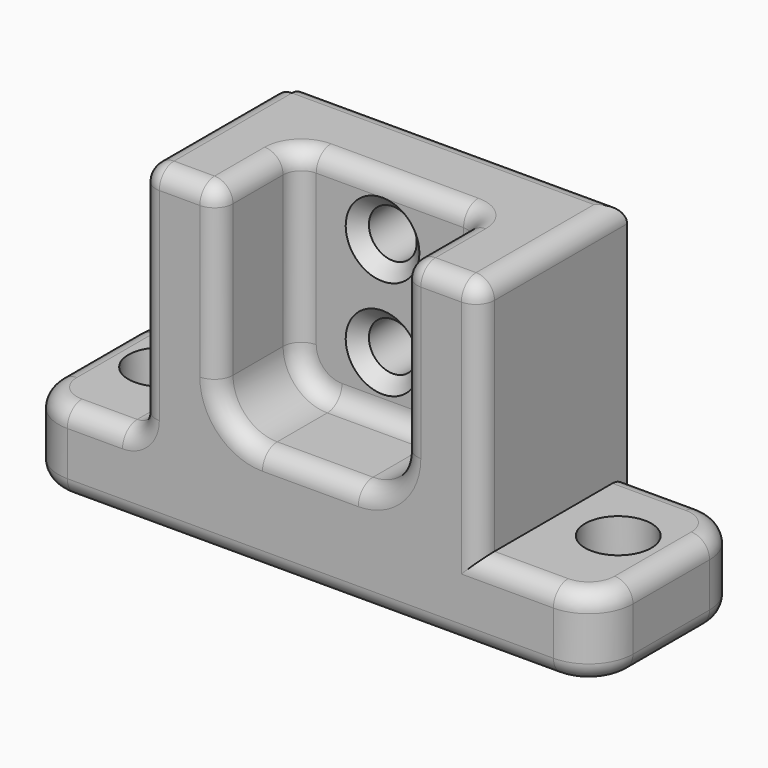
from build123d import *

# Parameters (mm, degrees)
F0_W           = 156
F0_H           = 50
F1_DEPTH       = 87
F2_W           = 32
F2_H           = 65
F3_DEPTH       = 50
F4_W           = 50
F4_H           = 58
F5_DEPTH       = 27
F7_D           = 13
F7_CBORE_D     = 18
F7_CBORE_DEPTH = 10
F9_D           = 13
F9_CSINK_D     = 20
F9_CSINK_ANGLE = 90
F10_R          = 12
F11_T1_DEPTH   = 46
F11_T3_DEPTH   = 26
F11_T5_DEPTH   = 50
F11_T8_ANGLE   = 90
F11_T10_ANGLE  = 90
F11_T11_DEPTH  = 57.5
F11_T13_DEPTH  = 28.5
F11_T15_DEPTH  = 46
F11_T17_DEPTH  = 75
F11_T19_DEPTH  = 117
F11_T21_DEPTH  = 132
F11_T23_DEPTH  = 20
F11_T25_DEPTH  = 60
F11_T27_DEPTH  = 58.5
F11_T29_DEPTH  = 26
F11_T31_DEPTH  = 26
F11_S35_W      = 5
F11_S35_H      = 5
F11_T36_DEPTH  = 5
F11_T40_ANGLE  = 90
F11_T42_ANGLE  = 90
F11_T44_ANGLE  = 90
F11_T46_ANGLE  = 90
F11_T48_ANGLE  = 90
F11_T50_ANGLE  = 90
F11_T52_ANGLE  = 90
F11_T54_ANGLE  = 90
F11_T59_DEPTH  = 72.5
F11_T63_DEPTH  = 32.5
F11_T66_DEPTH  = 17
F11_T68_DEPTH  = 40
F11_T70_DEPTH  = 15
F11_T72_DEPTH  = 55
F11_T74_DEPTH  = 26
F11_S78_W      = 5
F11_S78_H      = 5
F11_T79_DEPTH  = 5
F11_S84_W      = 5
F11_S84_H      = 5
F11_T85_DEPTH  = 5
F11_S90_W      = 5
F11_S90_H      = 5
F11_T91_DEPTH  = 5
F11_S96_W      = 5
F11_S96_H      = 5
F11_T97_DEPTH  = 5
F11_T101_ANGLE = 90
F11_T103_ANGLE = 90
F11_T105_ANGLE = 90
F11_T107_ANGLE = 90
F11_T109_ANGLE = 90
F11_T111_ANGLE = 90


# Not quite as in the source:
# - a fillet or chamfer that OpenCascade refuses, or shapes differently, is made with other operations: its cross-section is extruded or revolved along the edge and cut away or added


with BuildPart() as f1:
    # F0 (on Top) → F1 (new body)
    with BuildSketch(Plane.XY):
        with Locations((78, 25)):
            Rectangle(F0_W, F0_H)
    extrude(amount=F1_DEPTH)

    # F2 (on face) → F3 (cut, through all)
    with BuildSketch(Plane.XZ):
        with Locations((16, 54.5)):
            Rectangle(F2_W, F2_H)
        with Locations((140, 54.5)):
            Rectangle(F2_W, F2_H)
    extrude(amount=-F3_DEPTH, mode=Mode.SUBTRACT)

    # F4 (on face) → F5 (cut)
    with BuildSketch(Plane.XZ):
        with Locations((78, 58)):
            Rectangle(F4_W, F4_H)
    extrude(amount=-F5_DEPTH, mode=Mode.SUBTRACT)

    # F7 (through all)
    with Locations(Plane.XY.offset(22)):
        with Locations((16, 27), (140, 27)):
            CounterBoreHole(F7_D / 2, F7_CBORE_D / 2, F7_CBORE_DEPTH)

    # F9 (through all)
    with Locations(Plane.XZ.offset(-27)):
        with Locations((76, 72), (76, 45)):
            CounterSinkHole(F9_D / 2, F9_CSINK_D / 2, counter_sink_angle=F9_CSINK_ANGLE)

    # F10
    f10_edges = [f1.edges().sort_by_distance(p)[0] for p in [
        (53, 13.5, 29),
        (103, 13.5, 29),
        (0, 0, 11),
        (0, 50, 11),
        (156, 50, 11),
        (156, 0, 11),
    ]]
    fillet(f10_edges, radius=F10_R)

    # F11: fillet of radius 5 on 45 edges, made by hand

    # F11_s2 → F11_t1 (join)
    with BuildSketch(Plane.XY.offset(41)):
        with BuildLine():
            ThreePointArc((53, 22), (54.4644660941, 25.5355339059), (58, 27))
            Line((58, 27), (53, 27))
            Line((53, 27), (53, 22))
        make_face()
        with BuildLine():
            ThreePointArc((103, 22), (101.5355339059, 25.5355339059), (98, 27))
            Line((98, 27), (103, 27))
            Line((103, 27), (103, 22))
        make_face()
    extrude(amount=F11_T1_DEPTH)

    # F11_s4 → F11_t3 (join)
    with BuildSketch(Plane.YZ.offset(65)):
        with BuildLine():
            ThreePointArc((22, 29), (25.5355339059, 30.4644660941), (27, 34))
            Line((27, 34), (27, 29))
            Line((27, 29), (22, 29))
        make_face()
    extrude(amount=F11_T3_DEPTH)

    # F11_s6 → F11_t5 (join)
    with BuildSketch(Plane.XZ.offset(-50)):
        with BuildLine():
            ThreePointArc((27, 22), (30.5355339059, 23.4644660941), (32, 27))
            Line((32, 27), (32, 22))
            Line((32, 22), (27, 22))
        make_face()
    extrude(amount=F11_T5_DEPTH)

    # F11_s7 → F11_t8 (revolve)
    with BuildSketch(Plane.YZ.offset(65)):
        with BuildLine():
            ThreePointArc((22, 29), (25.5355339059, 30.4644660941), (27, 34))
            Line((27, 34), (27, 29))
            Line((27, 29), (22, 29))
        make_face()
    revolve(axis=Axis((65, 27, 41), (0, 1, 0)), revolution_arc=F11_T8_ANGLE)

    # F11_s9 → F11_t10 (revolve)
    with BuildSketch(Plane.XY.offset(41)):
        with BuildLine():
            ThreePointArc((103, 22), (101.5355339059, 25.5355339059), (98, 27))
            Line((98, 27), (103, 27))
            Line((103, 27), (103, 22))
        make_face()
    revolve(axis=Axis((91, 27, 41), (0, 1, 0)), revolution_arc=F11_T10_ANGLE)

    # F11_s12 → F11_t11 (cut)
    with BuildSketch(Plane.XZ.offset(-62.5)):
        with BuildLine():
            ThreePointArc((124, 82), (122.5355339059, 85.5355339059), (119, 87))
            Line((119, 87), (124, 87))
            Line((124, 87), (124, 82))
        make_face()
    extrude(amount=F11_T11_DEPTH, mode=Mode.SUBTRACT)

    # F11_s14 → F11_t13 (cut)
    with BuildSketch(Plane.YZ.offset(90.5)):
        with BuildLine():
            ThreePointArc((0, 82), (1.4644660941, 85.5355339059), (5, 87))
            Line((5, 87), (0, 87))
            Line((0, 87), (0, 82))
        make_face()
    extrude(amount=F11_T13_DEPTH, mode=Mode.SUBTRACT)

    # F11_s16 → F11_t15 (cut)
    with BuildSketch(Plane.YZ.offset(19.5)):
        with BuildLine():
            ThreePointArc((0, 82), (1.4644660941, 85.5355339059), (5, 87))
            Line((5, 87), (0, 87))
            Line((0, 87), (0, 82))
        make_face()
    extrude(amount=F11_T15_DEPTH, mode=Mode.SUBTRACT)

    # F11_s18 → F11_t17 (cut)
    with BuildSketch(Plane.XZ.offset(-62.5)):
        with BuildLine():
            ThreePointArc((32, 82), (33.4644660941, 85.5355339059), (37, 87))
            Line((37, 87), (32, 87))
            Line((32, 87), (32, 82))
        make_face()
    extrude(amount=F11_T17_DEPTH, mode=Mode.SUBTRACT)

    # F11_s20 → F11_t19 (cut)
    with BuildSketch(Plane.YZ.offset(19.5)):
        with BuildLine():
            ThreePointArc((50, 82), (48.5355339059, 85.5355339059), (45, 87))
            Line((45, 87), (50, 87))
            Line((50, 87), (50, 82))
        make_face()
    extrude(amount=F11_T19_DEPTH, mode=Mode.SUBTRACT)

    # F11_s22 → F11_t21 (cut)
    with BuildSketch(Plane.YZ.offset(12)):
        with BuildLine():
            ThreePointArc((5, 0), (1.4644660941, 1.4644660941), (0, 5))
            Line((0, 5), (0, 0))
            Line((0, 0), (5, 0))
        make_face()
        with BuildLine():
            ThreePointArc((45, 0), (48.5355339059, 1.4644660941), (50, 5))
            Line((50, 5), (50, 0))
            Line((50, 0), (45, 0))
        make_face()
    extrude(amount=F11_T21_DEPTH, mode=Mode.SUBTRACT)

    # F11_s24 → F11_t23 (cut)
    with BuildSketch(Plane.YZ.offset(124)):
        with BuildLine():
            ThreePointArc((0, 17), (1.4644660941, 20.5355339059), (5, 22))
            Line((5, 22), (0, 22))
            Line((0, 22), (0, 17))
        make_face()
        with BuildLine():
            ThreePointArc((50, 17), (48.5355339059, 20.5355339059), (45, 22))
            Line((45, 22), (50, 22))
            Line((50, 22), (50, 17))
        make_face()
    extrude(amount=F11_T23_DEPTH, mode=Mode.SUBTRACT)

    # F11_s26 → F11_t25 (cut)
    with BuildSketch(Plane.XY.offset(22)):
        with BuildLine():
            ThreePointArc((119, 0), (122.5355339059, 1.4644660941), (124, 5))
            Line((124, 5), (124, 0))
            Line((124, 0), (119, 0))
        make_face()
    extrude(amount=F11_T25_DEPTH, mode=Mode.SUBTRACT)

    # F11_s28 → F11_t27 (cut)
    with BuildSketch(Plane.XY.offset(41)):
        with BuildLine():
            ThreePointArc((48, 0), (51.5355339059, 1.4644660941), (53, 5))
            Line((53, 5), (53, 0))
            Line((53, 0), (48, 0))
        make_face()
        with BuildLine():
            ThreePointArc((108, 0), (104.4644660941, 1.4644660941), (103, 5))
            Line((103, 5), (103, 0))
            Line((103, 0), (108, 0))
        make_face()
    extrude(amount=F11_T27_DEPTH, mode=Mode.SUBTRACT)

    # F11_s30 → F11_t29 (cut)
    with BuildSketch(Plane.YZ.offset(65)):
        with BuildLine():
            ThreePointArc((0, 24), (1.4644660941, 27.5355339059), (5, 29))
            Line((5, 29), (0, 29))
            Line((0, 29), (0, 24))
        make_face()
    extrude(amount=F11_T29_DEPTH, mode=Mode.SUBTRACT)

    # F11_s32 → F11_t31 (cut)
    with BuildSketch(Plane.XZ.offset(-38)):
        with BuildLine():
            ThreePointArc((0, 5), (1.4644660941, 1.4644660941), (5, 0))
            Line((5, 0), (0, 0))
            Line((0, 0), (0, 5))
        make_face()
        with BuildLine():
            ThreePointArc((151, 0), (154.5355339059, 1.4644660941), (156, 5))
            Line((156, 5), (156, 0))
            Line((156, 0), (151, 0))
        make_face()
        with BuildLine():
            ThreePointArc((156, 17), (154.5355339059, 20.5355339059), (151, 22))
            Line((151, 22), (156, 22))
            Line((156, 22), (156, 17))
        make_face()
    extrude(amount=F11_T31_DEPTH, mode=Mode.SUBTRACT)


with BuildPart() as f11_tool34:
    # F11_s35 → F11_t36 (new body)
    with BuildSketch(Plane.XY.offset(82)):
        with Locations((121.5, 2.5)):
            Rectangle(F11_S35_W, F11_S35_H)
    extrude(amount=F11_T36_DEPTH)

    # F11_s37 → F11_t38 (revolve, cut)
    with BuildSketch(Plane(origin=(119, 5, 82), x_dir=(-0.7071067812, 0.7071067812, 0), z_dir=(0.7071067812, 0.7071067812, 0))):
        with BuildLine():
            ThreePointArc((0, -5), (5, 0), (0, 5))
            Line((0, 5), (0, -5))
        make_face()
    revolve(axis=Axis((119, 5, 82), (0, 0, 1)), mode=Mode.SUBTRACT)


with BuildPart() as f1_1:
    add(f1.part)

    # F11_t33: cut F11_tool34
    add(f11_tool34.part, mode=Mode.SUBTRACT)

    # F11_s39 → F11_t40 (revolve, cut)
    with BuildSketch(Plane.YZ.offset(65)):
        with BuildLine():
            ThreePointArc((0, 24), (1.4644660941, 27.5355339059), (5, 29))
            Line((5, 29), (0, 29))
            Line((0, 29), (0, 24))
        make_face()
    revolve(axis=Axis((65, 0, 41), (0, 1, 0)), revolution_arc=F11_T40_ANGLE, mode=Mode.SUBTRACT)

    # F11_s41 → F11_t42 (revolve, cut)
    with BuildSketch(Plane.XY.offset(41)):
        with BuildLine():
            ThreePointArc((108, 0), (104.4644660941, 1.4644660941), (103, 5))
            Line((103, 5), (103, 0))
            Line((103, 0), (108, 0))
        make_face()
    revolve(axis=Axis((91, 0, 41), (0, 1, 0)), revolution_arc=F11_T42_ANGLE, mode=Mode.SUBTRACT)

    # F11_s43 → F11_t44 (revolve, cut)
    with BuildSketch(Plane.XZ.offset(-38)):
        with BuildLine():
            ThreePointArc((5, 0), (1.4644660941, 1.4644660941), (0, 5))
            Line((0, 5), (0, 0))
            Line((0, 0), (5, 0))
        make_face()
    revolve(axis=Axis((12, 38, 0), (0, 0, -1)), revolution_arc=F11_T44_ANGLE, mode=Mode.SUBTRACT)

    # F11_s45 → F11_t46 (revolve, cut)
    with BuildSketch(Plane.XZ.offset(-12)):
        with BuildLine():
            ThreePointArc((5, 0), (1.4644660941, 1.4644660941), (0, 5))
            Line((0, 5), (0, 0))
            Line((0, 0), (5, 0))
        make_face()
    revolve(axis=Axis((12, 12, 0), (0, 0, 1)), revolution_arc=F11_T46_ANGLE, mode=Mode.SUBTRACT)

    # F11_s47 → F11_t48 (revolve, cut)
    with BuildSketch(Plane.YZ.offset(144)):
        with BuildLine():
            ThreePointArc((45, 0), (48.5355339059, 1.4644660941), (50, 5))
            Line((50, 5), (50, 0))
            Line((50, 0), (45, 0))
        make_face()
    revolve(axis=Axis((144, 38, 0), (0, 0, -1)), revolution_arc=F11_T48_ANGLE, mode=Mode.SUBTRACT)

    # F11_s49 → F11_t50 (revolve, cut)
    with BuildSketch(Plane.YZ.offset(144)):
        with BuildLine():
            ThreePointArc((5, 0), (1.4644660941, 1.4644660941), (0, 5))
            Line((0, 5), (0, 0))
            Line((0, 0), (5, 0))
        make_face()
    revolve(axis=Axis((144, 12, 0), (0, 0, 1)), revolution_arc=F11_T50_ANGLE, mode=Mode.SUBTRACT)

    # F11_s51 → F11_t52 (revolve, cut)
    with BuildSketch(Plane.YZ.offset(144)):
        with BuildLine():
            ThreePointArc((50, 17), (48.5355339059, 20.5355339059), (45, 22))
            Line((45, 22), (50, 22))
            Line((50, 22), (50, 17))
        make_face()
    revolve(axis=Axis((144, 38, 22), (0, 0, -1)), revolution_arc=F11_T52_ANGLE, mode=Mode.SUBTRACT)

    # F11_s53 → F11_t54 (revolve, cut)
    with BuildSketch(Plane.YZ.offset(144)):
        with BuildLine():
            ThreePointArc((0, 17), (1.4644660941, 20.5355339059), (5, 22))
            Line((5, 22), (0, 22))
            Line((0, 22), (0, 17))
        make_face()
    revolve(axis=Axis((144, 12, 22), (0, 0, 1)), revolution_arc=F11_T54_ANGLE, mode=Mode.SUBTRACT)


with BuildPart() as f11_tool57:
    # F11_s58 → F11_t59 (new body)
    with BuildSketch(Plane.XY.offset(82)):
        with BuildLine():
            ThreePointArc((119, 0), (122.5355339059, 1.4644660941), (124, 5))
            Line((124, 5), (124, 0))
            Line((124, 0), (119, 0))
        make_face()
    extrude(amount=-F11_T59_DEPTH)

    split(bisect_by=Plane.XY.offset(22), keep=Keep.BOTTOM)


with BuildPart() as f11_tool61:
    # F11_s62 → F11_t63 (new body)
    with BuildSketch(Plane.YZ.offset(111.5)):
        with BuildLine():
            ThreePointArc((0, 17), (1.4644660941, 20.5355339059), (5, 22))
            Line((5, 22), (0, 22))
            Line((0, 22), (0, 17))
        make_face()
    extrude(amount=F11_T63_DEPTH)

    split(bisect_by=Plane.YZ.offset(124), keep=Keep.BOTTOM)


with BuildPart() as f11_tool57_1:
    add(f11_tool57.part)

    # F11_t65: intersect F11_tool61
    add(f11_tool61.part, mode=Mode.INTERSECT)


with BuildPart() as f1_2:
    add(f1_1.part)

    # F11_t55: cut F11_tool57
    add(f11_tool57_1.part, mode=Mode.SUBTRACT)

    # F11_s67 → F11_t66 (cut)
    with BuildSketch(Plane.XZ.offset(-22)):
        with BuildLine():
            ThreePointArc((108, 87), (104.4644660941, 85.5355339059), (103, 82))
            Line((103, 82), (103, 87))
            Line((103, 87), (108, 87))
        make_face()
        with BuildLine():
            ThreePointArc((48, 87), (51.5355339059, 85.5355339059), (53, 82))
            Line((53, 82), (53, 87))
            Line((53, 87), (48, 87))
        make_face()
    extrude(amount=F11_T66_DEPTH, mode=Mode.SUBTRACT)

    # F11_s69 → F11_t68 (cut)
    with BuildSketch(Plane.YZ.offset(58)):
        with BuildLine():
            ThreePointArc((32, 87), (28.4644660941, 85.5355339059), (27, 82))
            Line((27, 82), (27, 87))
            Line((27, 87), (32, 87))
        make_face()
    extrude(amount=F11_T68_DEPTH, mode=Mode.SUBTRACT)

    # F11_s71 → F11_t70 (cut)
    with BuildSketch(Plane.YZ.offset(12)):
        with BuildLine():
            ThreePointArc((0, 17), (1.4644660941, 20.5355339059), (5, 22))
            Line((5, 22), (0, 22))
            Line((0, 22), (0, 17))
        make_face()
        with BuildLine():
            ThreePointArc((50, 17), (48.5355339059, 20.5355339059), (45, 22))
            Line((45, 22), (50, 22))
            Line((50, 22), (50, 17))
        make_face()
    extrude(amount=F11_T70_DEPTH, mode=Mode.SUBTRACT)

    # F11_s73 → F11_t72 (cut)
    with BuildSketch(Plane.XY.offset(27)):
        with BuildLine():
            ThreePointArc((37, 0), (33.4644660941, 1.4644660941), (32, 5))
            Line((32, 5), (32, 0))
            Line((32, 0), (37, 0))
        make_face()
        with BuildLine():
            ThreePointArc((32, 45), (33.4644660941, 48.5355339059), (37, 50))
            Line((37, 50), (32, 50))
            Line((32, 50), (32, 45))
        make_face()
    extrude(amount=F11_T72_DEPTH, mode=Mode.SUBTRACT)

    # F11_s75 → F11_t74 (cut)
    with BuildSketch(Plane.XZ.offset(-38)):
        with BuildLine():
            ThreePointArc((0, 17), (1.4644660941, 20.5355339059), (5, 22))
            Line((5, 22), (0, 22))
            Line((0, 22), (0, 17))
        make_face()
    extrude(amount=F11_T74_DEPTH, mode=Mode.SUBTRACT)


with BuildPart() as f11_tool77:
    # F11_s78 → F11_t79 (new body)
    with BuildSketch(Plane.YZ.offset(37)):
        with Locations((47.5, 84.5)):
            Rectangle(F11_S78_W, F11_S78_H)
    extrude(amount=-F11_T79_DEPTH)

    # F11_s80 → F11_t81 (revolve, cut)
    with BuildSketch(Plane(origin=(37, 45, 82), x_dir=(0, -0.7071067812, -0.7071067812), z_dir=(0, 0.7071067812, -0.7071067812))):
        with BuildLine():
            ThreePointArc((0, -5), (5, 0), (0, 5))
            Line((0, 5), (0, -5))
        make_face()
    revolve(axis=Axis((37, 45, 82), (-1, 0, 0)), mode=Mode.SUBTRACT)


with BuildPart() as f1_3:
    add(f1_2.part)

    # F11_t76: cut F11_tool77
    add(f11_tool77.part, mode=Mode.SUBTRACT)


with BuildPart() as f11_tool83:
    # F11_s84 → F11_t85 (new body)
    with BuildSketch(Plane.XZ.offset(-5)):
        with Locations((34.5, 84.5)):
            Rectangle(F11_S84_W, F11_S84_H)
    extrude(amount=F11_T85_DEPTH)

    # F11_s86 → F11_t87 (revolve, cut)
    with BuildSketch(Plane(origin=(37, 5, 82), x_dir=(0.7071067812, 0, -0.7071067812), z_dir=(-0.7071067812, 0, -0.7071067812))):
        with BuildLine():
            ThreePointArc((0, -5), (5, 0), (0, 5))
            Line((0, 5), (0, -5))
        make_face()
    revolve(axis=Axis((37, 5, 82), (0, -1, 0)), mode=Mode.SUBTRACT)


with BuildPart() as f1_4:
    add(f1_3.part)

    # F11_t82: cut F11_tool83
    add(f11_tool83.part, mode=Mode.SUBTRACT)


with BuildPart() as f11_tool89:
    # F11_s90 → F11_t91 (new body)
    with BuildSketch(Plane.XY.offset(82)):
        with Locations((50.5, 2.5)):
            Rectangle(F11_S90_W, F11_S90_H)
    extrude(amount=F11_T91_DEPTH)

    # F11_s92 → F11_t93 (revolve, cut)
    with BuildSketch(Plane(origin=(48, 5, 82), x_dir=(-0.7071067812, 0.7071067812, 0), z_dir=(0.7071067812, 0.7071067812, 0))):
        with BuildLine():
            ThreePointArc((0, -5), (5, 0), (0, 5))
            Line((0, 5), (0, -5))
        make_face()
    revolve(axis=Axis((48, 5, 82), (0, 0, 1)), mode=Mode.SUBTRACT)


with BuildPart() as f1_5:
    add(f1_4.part)

    # F11_t88: cut F11_tool89
    add(f11_tool89.part, mode=Mode.SUBTRACT)


with BuildPart() as f11_tool95:
    # F11_s96 → F11_t97 (new body)
    with BuildSketch(Plane.XY.offset(82)):
        with Locations((105.5, 2.5)):
            Rectangle(F11_S96_W, F11_S96_H)
    extrude(amount=F11_T97_DEPTH)

    # F11_s98 → F11_t99 (revolve, cut)
    with BuildSketch(Plane(origin=(108, 5, 82), x_dir=(0.7071067812, 0.7071067812, 0), z_dir=(0.7071067812, -0.7071067812, 0))):
        with BuildLine():
            ThreePointArc((0, -5), (5, 0), (0, 5))
            Line((0, 5), (0, -5))
        make_face()
    revolve(axis=Axis((108, 5, 82), (0, 0, 1)), mode=Mode.SUBTRACT)


with BuildPart() as f1_6:
    add(f1_5.part)

    # F11_t94: cut F11_tool95
    add(f11_tool95.part, mode=Mode.SUBTRACT)

    # F11_s100 → F11_t101 (revolve, cut)
    with BuildSketch(Plane.XZ.offset(-38)):
        with BuildLine():
            ThreePointArc((0, 17), (1.4644660941, 20.5355339059), (5, 22))
            Line((5, 22), (0, 22))
            Line((0, 22), (0, 17))
        make_face()
    revolve(axis=Axis((12, 38, 22), (0, 0, -1)), revolution_arc=F11_T101_ANGLE, mode=Mode.SUBTRACT)

    # F11_s102 → F11_t103 (revolve, cut)
    with BuildSketch(Plane.XZ.offset(-12)):
        with BuildLine():
            ThreePointArc((5, 22), (1.4644660941, 20.5355339059), (0, 17))
            Line((0, 17), (0, 22))
            Line((0, 22), (5, 22))
        make_face()
    revolve(axis=Axis((12, 12, 22), (0, 0, 1)), revolution_arc=F11_T103_ANGLE, mode=Mode.SUBTRACT)

    # F11_s104 → F11_t105 (revolve, cut)
    with BuildSketch(Plane.YZ.offset(27)):
        with BuildLine():
            ThreePointArc((45, 22), (48.5355339059, 20.5355339059), (50, 17))
            Line((50, 17), (50, 22))
            Line((50, 22), (45, 22))
        make_face()
    revolve(axis=Axis((27, 50, 27), (0, -1, 0)), revolution_arc=F11_T105_ANGLE, mode=Mode.SUBTRACT)

    # F11_s106 → F11_t107 (revolve, cut)
    with BuildSketch(Plane.YZ.offset(27)):
        with BuildLine():
            ThreePointArc((0, 17), (1.4644660941, 20.5355339059), (5, 22))
            Line((5, 22), (0, 22))
            Line((0, 22), (0, 17))
        make_face()
    revolve(axis=Axis((27, 0, 27), (0, -1, 0)), revolution_arc=F11_T107_ANGLE, mode=Mode.SUBTRACT)

    # F11_s108 → F11_t109 (revolve, cut)
    with BuildSketch(Plane.XZ.offset(-22)):
        with BuildLine():
            ThreePointArc((48, 87), (51.5355339059, 85.5355339059), (53, 82))
            Line((53, 82), (53, 87))
            Line((53, 87), (48, 87))
        make_face()
    revolve(axis=Axis((58, 22, 87), (0, 0, -1)), revolution_arc=F11_T109_ANGLE, mode=Mode.SUBTRACT)

    # F11_s110 → F11_t111 (revolve, cut)
    with BuildSketch(Plane.XZ.offset(-22)):
        with BuildLine():
            ThreePointArc((108, 87), (104.4644660941, 85.5355339059), (103, 82))
            Line((103, 82), (103, 87))
            Line((103, 87), (108, 87))
        make_face()
    revolve(axis=Axis((98, 22, 87), (0, 0, 1)), revolution_arc=F11_T111_ANGLE, mode=Mode.SUBTRACT)


solid = f1_6.part
